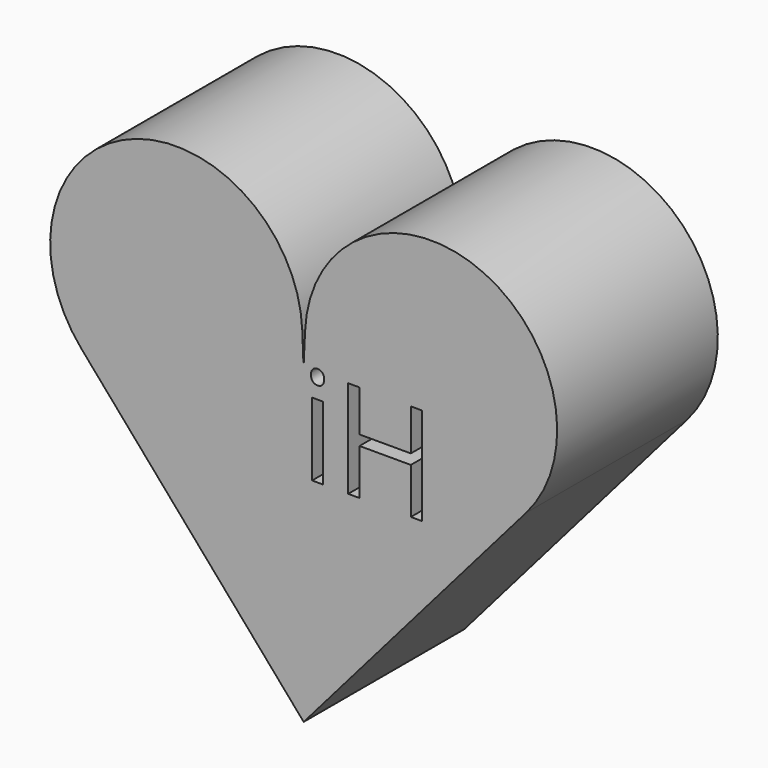
from build123d import *

# Parameters (mm, degrees)
F1_DEPTH     = 36.576
F2_TEXT_SIZE = 24.8457149913
F3_DEPTH     = 42.418


# Not quite as in the source:
# - Text() gives the source's letters only with a copy of the font that has no kerning and outlines rounded to 1/6400 em; it was checked with that copy


with BuildPart() as f1:
    # F0 (on Front) → F1 (new body)
    with BuildSketch(Plane.XZ):
        with BuildLine():
            ThreePointArc((-0.2564353649, 38.3396146313), (-31.666863108, 58.7703531137), (-40.5545302208, 22.3692622066))
            Line((-40.5545302208, 22.3692622066), (0, -24.3828333914))
            Line((0, -24.3828333914), (40.5545302208, 22.3692622066))
            ThreePointArc((40.5545302208, 22.3692622066), (31.6715975612, 58.7684762169), (0.2568460028, 38.3497921817))
            Line((0.2568460028, 38.3497921817), (-0.0226190738, 32.5124631451))
            Line((-0.0226190738, 32.5124631451), (-0.2564353649, 38.3396146313))
        make_face()
    extrude(amount=F1_DEPTH)

    # F2 (on face) → F3 (cut)
    with BuildSketch(Plane(origin=(0, 0, 0), x_dir=(-1, 0, 0), z_dir=(0, 1, 0))):
        with Locations((-24.0152534097, 14.8257426918)):
            Text('Hi', F2_TEXT_SIZE, font='Open Sans', text_align=(TextAlign.LEFT, TextAlign.BOTTOM))
    extrude(amount=-F3_DEPTH, mode=Mode.SUBTRACT)


solid = f1.part
